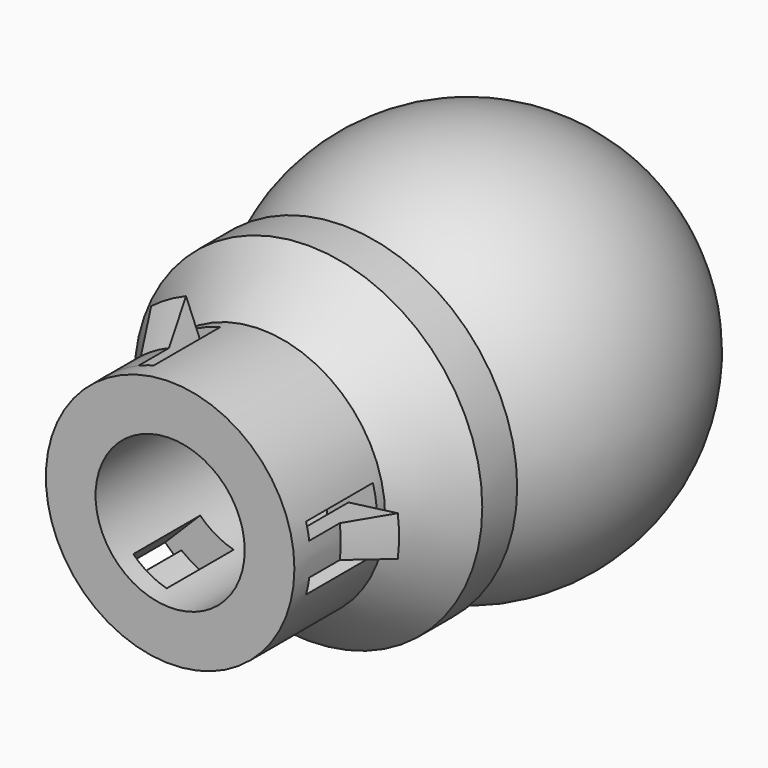
from build123d import *
from build123d import SkipClean  # not in build123d's __all__

# Parameters (mm, degrees)
F0_W            = 5
F0_H            = 4.387505004
F3_ANGLE_BACK   = 15
F3_ANGLE        = 30
F3_COPIES_COUNT = 3
F4_ANGLE_BACK   = 7.5
F4_ANGLE        = 15
F4_COPIES_COUNT = 3


# Not quite as in the source:
# - a pattern or mirror of a feature is missing from the dataset's text; its kind, count and spacing are read off the source's solid


with BuildPart() as f1:
    # F0 (on Top) → F1 (revolve)
    with BuildSketch(Plane.XY):
        with BuildLine():
            ThreePointArc((12.5, 21.7588313682), (18.8712731409, 43.9951507913), (0, 57.3713263642))
            Line((0, 57.3713263642), (0, 52.3713263642))
            ThreePointArc((0, 52.3713263642), (14.4888873943, 41.2536120408), (7.5, 24.3809453075))
            Line((7.5, 24.3809453075), (7.5, 18.8308301465))
            ThreePointArc((7.5, 18.8308301465), (10.1065967461, 20.1128008707), (12.5, 21.7588313682))
        make_face()
        with BuildLine():
            Line((12.5, 17.3713263642), (12.5, 21.7588313682))
            ThreePointArc((12.5, 21.7588313682), (10.1065967461, 20.1128008707), (7.5, 18.8308301465))
            Line((7.5, 18.8308301465), (7.5, 0))
            Line((7.5, 0), (12.5, 0))
            Line((12.5, 0), (12.5, 11.4125584013))
            Line((12.5, 11.4125584013), (12.5, 17.3713263642))
        make_face()
        with Locations((15, 19.5650788662)):
            Rectangle(F0_W, F0_H)
        Polygon((17.5, 17.3713263642), (12.5, 17.3713263642), (12.5, 11.4125584013), align=None)
    revolve(axis=Axis((0, 26.1856631821, 0), (0, 1, 0)))

    # F2 (on Top) → F3 (revolve, cut)
    with BuildSketch(Plane.XY, mode=Mode.PRIVATE) as f3_sk:
        Polygon((7.5, 10.4125584013), (7.5, 2), (10.5, 2), (10.5, 9.4125584013), (12.5, 9.4125584013), (12.5, 10.4125584013), align=None)
        Polygon((10.5, 2), (12.5, 2), (12.5, 5.8372976235), (12.5, 9.4125584013), (10.5, 9.4125584013), align=None)
    f3 = revolve(f3_sk.sketch.rotate(Axis((0, 0, 0), (0, -1, 0)), -F3_ANGLE_BACK), axis=Axis((0, 0, 0), (0, -1, 0)), revolution_arc=F3_ANGLE, mode=Mode.SUBTRACT)

    # F3_copies: F3 ×3 about axis
    f3_copies_axis = Axis((0, 0, 0), (0, 1, 0))
    for i in range(1, F3_COPIES_COUNT):
        add(f3.rotate(f3_copies_axis, i * 360 / F3_COPIES_COUNT), clean=False, mode=Mode.SUBTRACT)

    # F2 (on Top) → F4 (revolve)
    with BuildSketch(Plane.XY, mode=Mode.PRIVATE) as f4_sk:
        Polygon((12.5, 9.4125584013), (12.5, 5.8372976235), (15.5, 9.4125584013), align=None)
        Polygon((10.5, 2), (12.5, 2), (12.5, 5.8372976235), (12.5, 9.4125584013), (10.5, 9.4125584013), align=None)
    f4 = revolve(f4_sk.sketch.rotate(Axis((0, 0, 0), (0, 1, 0)), -F4_ANGLE_BACK), axis=Axis((0, 0, 0), (0, 1, 0)), revolution_arc=F4_ANGLE)

    # F4_copies: F4 ×3 about axis
    f4_copies_axis = Axis((0, 0, 0), (0, 1, 0))
    with SkipClean():  # cleaning this boolean's faces spoils the solid; the shape is the same uncleaned
        for i in range(1, F4_COPIES_COUNT):
            add(f4.rotate(f4_copies_axis, i * 360 / F4_COPIES_COUNT), clean=False)


solid = f1.part
